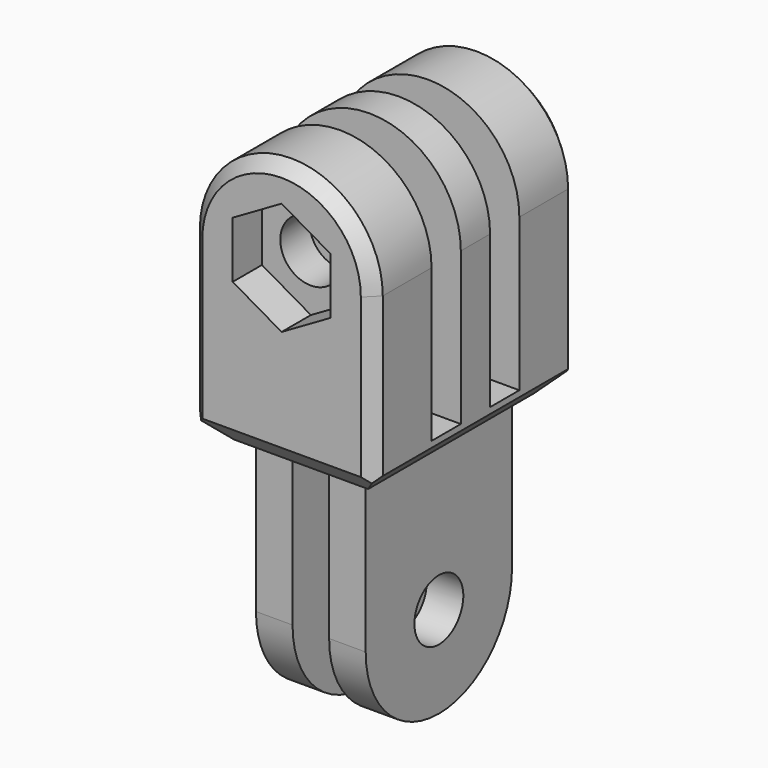
from build123d import *

# Parameters (mm, degrees)
F0_W      = 15
F0_H      = 21
F1_DEPTH  = 1.25
F2_W      = 15
F2_H      = 6
F2_H_2    = 3
F3_DEPTH  = 20
F4_W      = 3
F4_H      = 15
F5_DEPTH  = 20
F6_R      = 2.505
F7_DEPTH  = 25
F8_R      = 2.505
F9_DEPTH  = 25
F10_SIZE  = 2
F11_DEPTH = 3
F12_SIZE  = 2.7
F13_SIZE  = 1


with BuildPart() as f1:
    # F0 (on Top) → F1 (new body, symmetric)
    with BuildSketch(Plane.XY):
        Rectangle(F0_W, F0_H)
    extrude(amount=F1_DEPTH, both=True)

    # F2 (on face) → F3 (join)
    with BuildSketch(Plane.XY.offset(1.25)):
        with Locations((0, -7.5)):
            Rectangle(F2_W, F2_H)
        Rectangle(F2_W, F2_H_2)
        with Locations((0, 7.5)):
            Rectangle(F2_W, F2_H)
    extrude(amount=F3_DEPTH)

    # F4 (on face) → F5 (join)
    with BuildSketch(Plane(origin=(0, 0, -1.25), x_dir=(1, 0, 0), z_dir=(0, 0, -1))):
        with Locations((-3, 0)):
            Rectangle(F4_W, F4_H)
        with Locations((3, 0)):
            Rectangle(F4_W, F4_H)
    extrude(amount=F5_DEPTH)

    # F6 (on face) → F7 (cut)
    with BuildSketch(Plane.XZ.offset(10.5)):
        with BuildLine():
            ThreePointArc((0, 21.25), (5.3033008589, 19.0533008589), (7.5, 13.75))
            Line((7.5, 13.75), (7.5, 21.25))
            Line((7.5, 21.25), (0, 21.25))
        make_face()
        with BuildLine():
            ThreePointArc((-7.5, 13.75), (-5.3033008589, 19.0533008589), (0, 21.25))
            Line((0, 21.25), (-7.5, 21.25))
            Line((-7.5, 21.25), (-7.5, 13.75))
        make_face()
        with Locations((0, 13.75)):
            Circle(F6_R)
    extrude(amount=-F7_DEPTH, mode=Mode.SUBTRACT)

    # F8 (on face) → F9 (cut)
    with BuildSketch(Plane(origin=(-4.5, 0, 0), x_dir=(0, -1, 0), z_dir=(-1, 0, 0))):
        with BuildLine():
            Line((7.5, -21.25), (7.5, -13.75))
            ThreePointArc((7.5, -13.75), (5.3033008589, -19.0533008589), (0, -21.25))
            Line((0, -21.25), (7.5, -21.25))
        make_face()
        with BuildLine():
            ThreePointArc((0, -21.25), (-5.3033008589, -19.0533008589), (-7.5, -13.75))
            Line((-7.5, -13.75), (-7.5, -21.25))
            Line((-7.5, -21.25), (0, -21.25))
        make_face()
        with Locations((0, -13.75)):
            Circle(F8_R)
    extrude(amount=-F9_DEPTH, mode=Mode.SUBTRACT)

    # F10
    f10_edges = [f1.edges().sort_by_distance(p)[0] for p in [
        (-7.5, 0, -1.25),
        (0, 10.5, -1.25),
        (0, -10.5, -1.25),
        (7.5, 0, -1.25),
    ]]
    chamfer(f10_edges, length=F10_SIZE)

    # F6 (on face) → F11 (cut)
    with BuildSketch(Plane.XZ.offset(10.5)):
        Polygon((4.0080889509, 16.0684814631), (-0.0038193698, 18.3803475837), (-4.0119083207, 16.0618661206), (-4.0080889509, 11.4315185369), (0.0038193698, 9.1196524163), (4.0119083207, 11.4381338794), align=None)
        with Locations((0, 13.75)):
            Circle(F6_R, mode=Mode.SUBTRACT)
    extrude(amount=-F11_DEPTH, mode=Mode.SUBTRACT)

    # F12
    f12_edges = [f1.edges().sort_by_distance(p)[0] for p in [
        (-2.505, 10.5, 13.75),
    ]]
    chamfer(f12_edges, length=F12_SIZE)

    # F13
    f13_edges = [f1.edges().sort_by_distance(p)[0] for p in [
        (0, 10.5, 21.25),
        (7.5, 10.5, 7.25),
        (-7.5, 10.5, 7.25),
        (7.5, -10.5, 7.25),
        (-7.5, -10.5, 7.25),
        (0, -10.5, 21.25),
    ]]
    chamfer(f13_edges, length=F13_SIZE)


solid = f1.part
